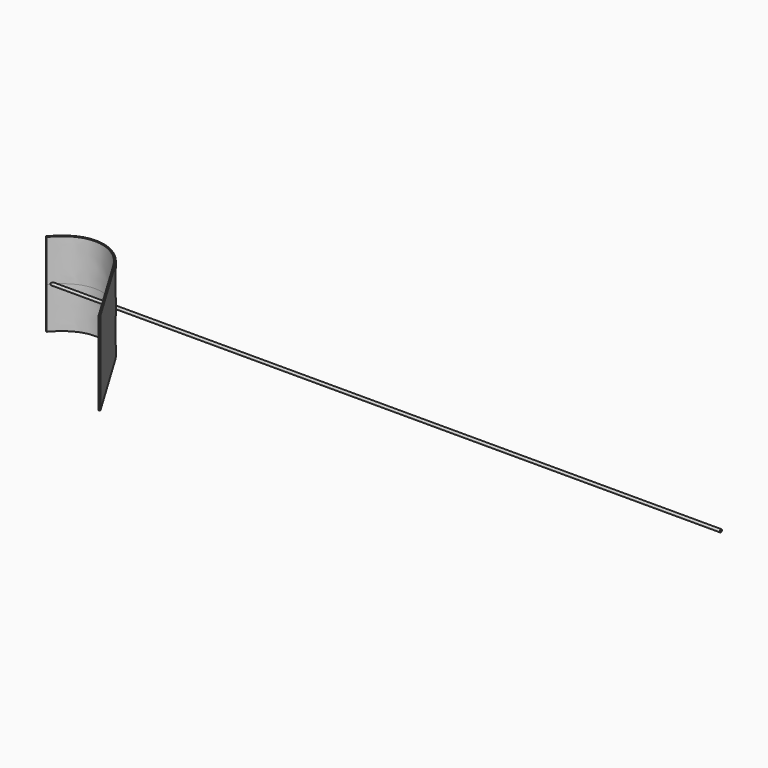
from build123d import *

# Parameters (mm, degrees)
F1_DEPTH      = 3
F3_R          = 0.1
F4_DEPTH      = 40
F4_DEPTH_BACK = 8.2


with BuildPart() as f1:
    # F0 (on Top) → F1 (new body, symmetric)
    with BuildSketch(Plane.XY):
        with BuildLine():
            Line((-8.3363476084, 5.7012820817), (-8.2600094956, 5.6366872481))
            add(Edge.make_bspline(
                [(-8.2600094956, 5.6366872481), (-6.3820579089, 7.8560486436), (-4.1340692605, 6.8935410618), (-3.2040320802, 5.3427084349)],
                knots=[0, 0, 0, 0, 5.064516874, 5.064516874, 5.064516874, 5.064516874], degree=3))
            Line((-3.2040320802, 5.3427084349), (0, 0))
            Line((0, 0), (0.0857605715, 0.0514307726))
            Line((0.0857605715, 0.0514307726), (-3.1182715087, 5.3941392075))
            add(Edge.make_bspline(
                [(-8.3363476084, 5.7012820817), (-7.858202706, 6.2663532717), (-6.8462270118, 7.0009139545), (-5.3268128413, 7.1244076412), (-4.0041163546, 6.5138933081), (-3.3575728268, 5.7931730307), (-3.1182715087, 5.3941392075)],
                knots=[0, 0, 0, 0, 0.25, 0.5, 0.75, 1, 1, 1, 1], degree=3))
        make_face()
    extrude(amount=F1_DEPTH, both=True)


with BuildPart() as f4:
    # F3 (on offset) → F4 (new body, two sides)
    with BuildSketch(Plane.YZ) as f4_sk:
        with Locations((5.8941392075, 0)):
            Circle(F3_R)
    extrude(amount=F4_DEPTH)
    extrude(f4_sk.sketch, amount=-F4_DEPTH_BACK)


solid = Compound([f1.part, f4.part])
